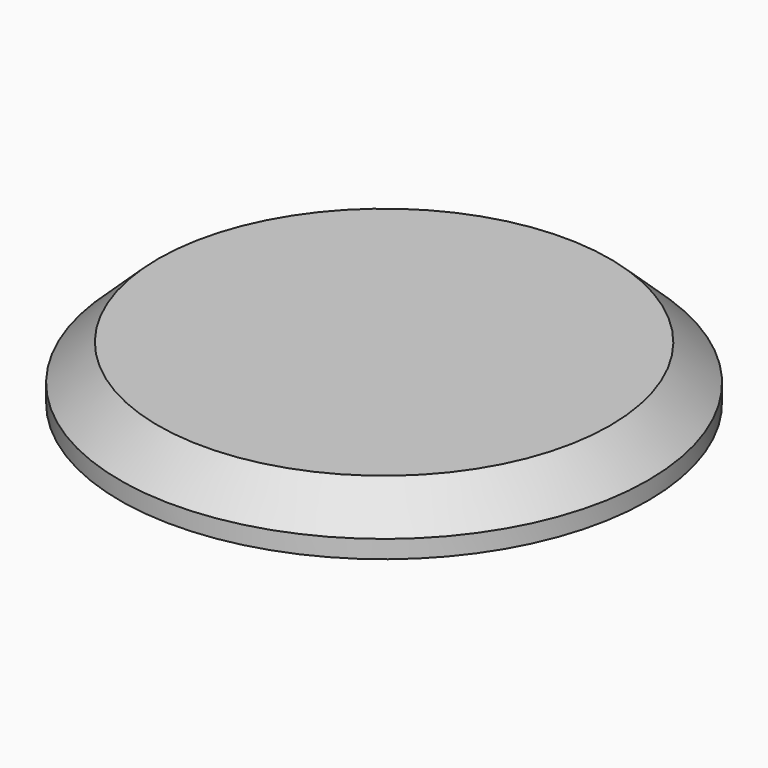
from build123d import *

# Parameters (mm, degrees)
F3_R     = 14.7507803317
F4_DEPTH = 1
F7_R     = 12.623224735


# Not quite as in the source:
# - the program builds the solid bodies; features that only make, move or delete a surface that nothing else refers to are left out


with BuildPart() as f4:
    # F3 (on face) → F4 (new body)
    with BuildSketch(Plane(origin=(0, 0, -15), x_dir=(1, 0, 0), z_dir=(0, 0, -1))):
        Circle(F3_R)
    extrude(amount=F4_DEPTH)

    # F3 (on face) → F8 section 0
    with BuildSketch(Plane(origin=(0, 0, -15), x_dir=(1, 0, 0), z_dir=(0, 0, -1))):
        Circle(F3_R)
    # F7 (on offset) → F8 section 1
    with BuildSketch(Plane(origin=(0, 0, -13), x_dir=(1, 0, 0), z_dir=(0, 0, -1))):
        Circle(F7_R)
    loft()


solid = f4.part
